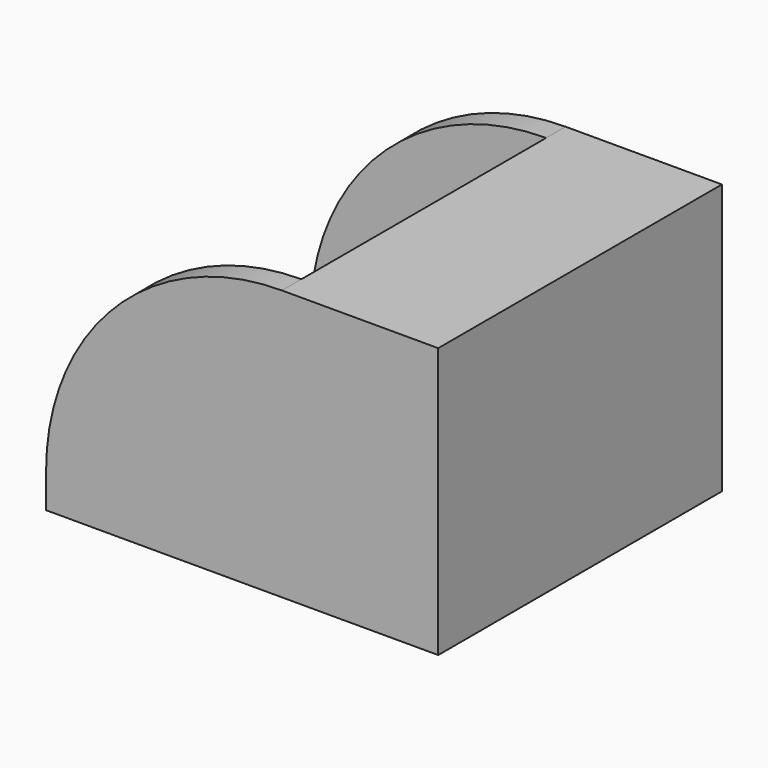
from build123d import *

# Parameters (mm, degrees)
F0_W     = 36.8659496307
F0_H     = 33.33741799
F1_DEPTH = 25.4
F2_R     = 22.1712758518
F3_T     = 2.286


# Not quite as in the source:
# - a shell that OpenCascade refuses in one call is made with other operations: the cavity is built on its own and cut out


with BuildPart() as f1:
    # F0 (on Top) → F1 (new body)
    with BuildSketch(Plane.XY):
        Rectangle(F0_W, F0_H)
    extrude(amount=F1_DEPTH)

    # F2
    f2_edges = [f1.edges().sort_by_distance(p)[0] for p in [
        (-18.432975, 0, 25.4),
    ]]
    fillet(f2_edges, radius=F2_R)

    # F3: shell of thickness 2.286, made by hand


with BuildPart() as f3_core1:
    # F3_t2: copy of F1
    add(f1.part)

    # the walls: a layer under each face that stays
    f3_faces = [f3_core1.faces().sort_by_distance(p)[0] for p in [
        (0, 16.668708995, 12.7),
        (-18.4329748154, 0, 1.6143620741),
        (0, 0, 0),
        (11.0856379259, 0, 25.4),
        (18.4329748154, 0, 12.7),
        (0, -16.668708995, 12.7),
    ]]
    thicken(f3_faces, amount=-F3_T, mode=Mode.SUBTRACT)


with BuildPart() as f1_1:
    add(f1.part)

    # what is left inside the walls is the cavity
    f3_cavity = [f3_core1.part.solids().sort_by_distance(p)[0] for p in [
        (-11.922994, 4.794236, 18.890019),
    ]]
    add(f3_cavity, mode=Mode.SUBTRACT)


solid = f1_1.part
